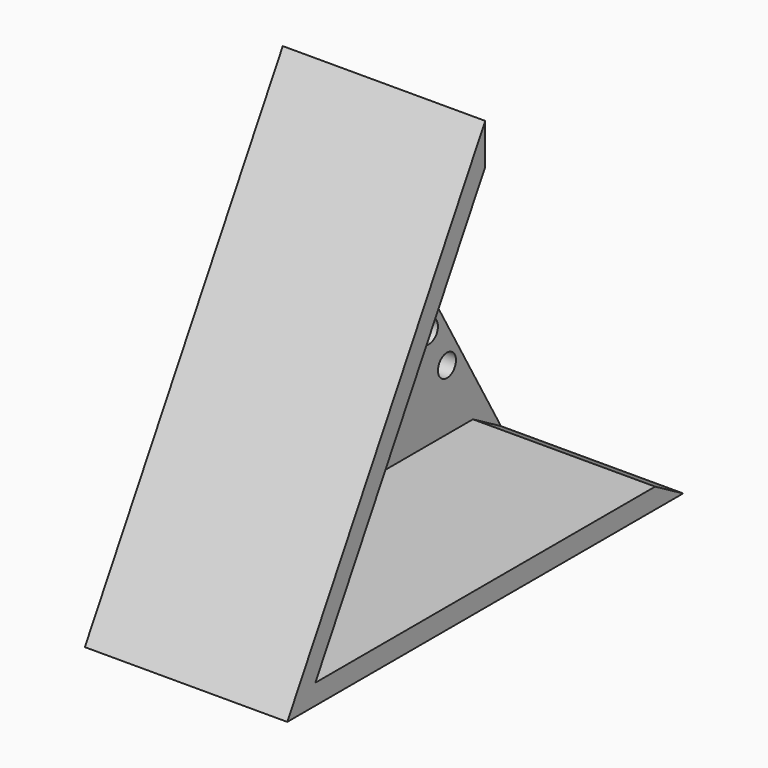
from build123d import *

# Parameters (mm, degrees)
F1_DEPTH = 45
F2_T     = -4.5
F4_D     = 5
F4_DEPTH = 12
F4_TIP   = 1.5021515476
F6_DEPTH = 40.5


with BuildPart() as f1:
    # F0 (on Right) → F1 (new body)
    with BuildSketch(Plane.YZ):
        Polygon((-46.7345683003, 84.126270037), (-101.7345683003, -11.1365243793), (8.2654316997, -11.1365243793), align=None)
    extrude(amount=F1_DEPTH)

    # F2
    f2_openings = [f1.faces().sort_by_distance(p)[0] for p in [
        (45, -46.734568, 20.61774),
    ]]
    offset(amount=F2_T, openings=f2_openings)

    # F4
    with Locations(Plane(origin=(0, 0, 0), x_dir=(0, -1, 0), z_dir=(-1, 0, 0))):
        with Locations((36.7409650803, 58.8168415093), (31.7409650803, 50.1565874715), (26.7409650803, 41.4963334336), (21.7409650803, 32.8360793958), (16.7409650803, 24.1758253579), (11.7409650803, 15.5155713201), (6.7409650803, 6.8553172823)):
            Hole(F4_D / 2, depth=F4_DEPTH)
            with Locations((0, 0, -(F4_DEPTH + F4_TIP / 2))):  # 118° drill point
                Cone(0, F4_D / 2, F4_TIP, mode=Mode.SUBTRACT)

    # F5 (on face) → F6 (cut, symmetric)
    with BuildSketch(Plane.YZ.offset(45)):
        Polygon((-46.7345683003, 84.126270037), (-46.7345683003, 75.126270037), (0.4712030657, -6.6365243793), (8.2654316997, -11.1365243793), align=None)
    extrude(amount=F6_DEPTH, both=True, mode=Mode.SUBTRACT)


solid = f1.part
